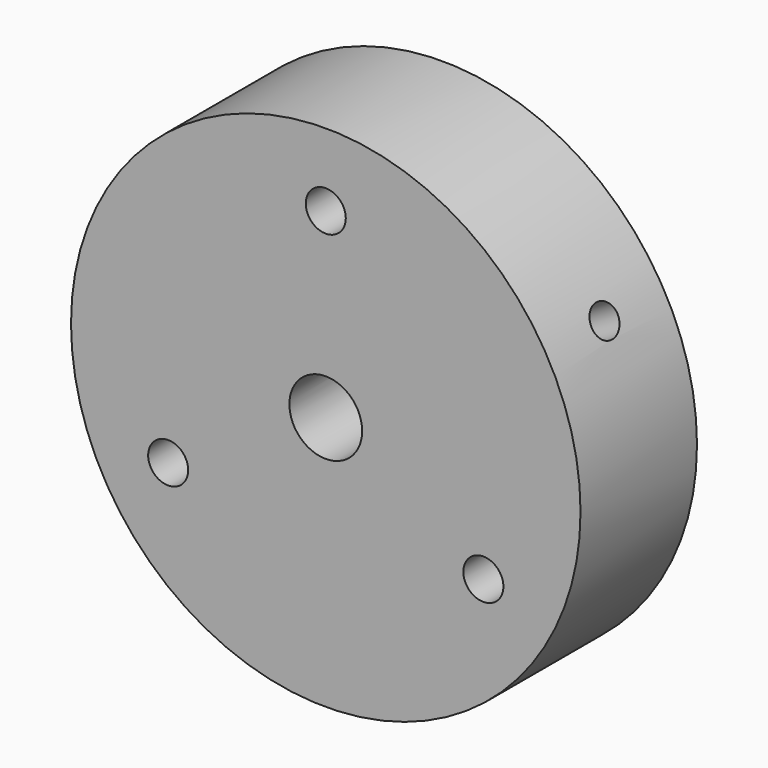
from build123d import *

# Parameters (mm, degrees)
F0_R     = 14
F0_R_2   = 1.1
F1_DEPTH = 8
F2_R     = 2
F3_DEPTH = 8.001
F6_R     = 0.875
F7_DEPTH = 19.125355653


# Not quite as in the source:
# - a pattern or mirror of a feature is missing from the dataset's text; its kind, count and spacing are read off the source's solid


with BuildPart() as f1:
    # F0 (on Front) → F1 (new body)
    with BuildSketch(Plane.XZ):
        Circle(F0_R)
        with Locations((-8.6602540378, -5)):
            Circle(F0_R_2, mode=Mode.SUBTRACT)
        with Locations((8.6602540378, -5)):
            Circle(F0_R_2, mode=Mode.SUBTRACT)
        with Locations((0, 10)):
            Circle(F0_R_2, mode=Mode.SUBTRACT)
    extrude(amount=F1_DEPTH)

    # F2 (on face) → F3 (cut, through all)
    with BuildSketch(Plane.XZ.offset(8)):
        Circle(F2_R)
    extrude(amount=-F3_DEPTH, mode=Mode.SUBTRACT)

    # F6 (on line) → F7 (cut, through all)
    with BuildSketch(Plane(origin=(0, 0, 0), x_dir=(0, 1, 0), z_dir=(0.8660254038, 0, -0.5))):
        with Locations((-4, 0)):
            Circle(F6_R)
    f7 = extrude(amount=-F7_DEPTH, mode=Mode.SUBTRACT)

    # F7_copies: F7 across plane
    add(f7.mirror(Plane(origin=(2e-05, 0, 0), x_dir=(-1e-06, 0, 1), z_dir=(1, 0, 1e-06))), mode=Mode.SUBTRACT)


solid = f1.part
